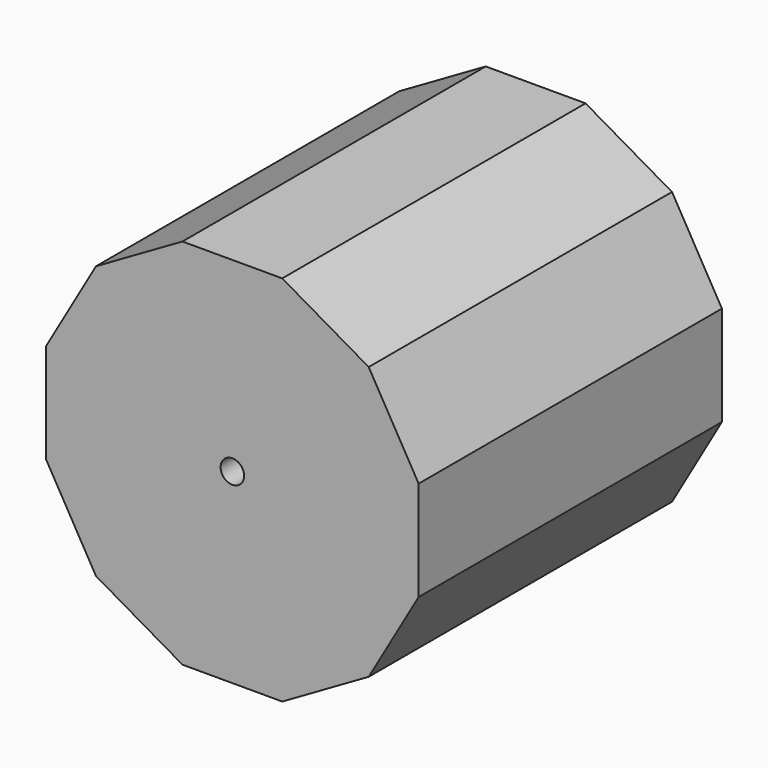
from build123d import *

# Parameters (mm, degrees)
F0_R     = 1.5694812218
F1_DEPTH = 50.8


# Not quite as in the source:
# - a feature names something its author has since deleted; it is built from what else it names


with BuildPart() as f1:
    # F0 (on Front) → F1 (new body)
    with BuildSketch(Plane.XZ):
        Polygon((6.6879468774, 24.9597575449), (-6.6879468774, 24.9597575449), (-18.2718106675, 18.2718106675), (-24.9597575449, 6.6879468774), (-24.9597575449, -6.6879468774), (-18.2718106675, -18.2718106675), (-6.6879468774, -24.9597575449), (6.6879468774, -24.9597575449), (18.2718106675, -18.2718106675), (24.9597575449, -6.6879468774), (24.9597575449, 6.6879468774), (18.2718106675, 18.2718106675), align=None)
        Circle(F0_R, mode=Mode.SUBTRACT)
    extrude(amount=F1_DEPTH)


solid = f1.part
